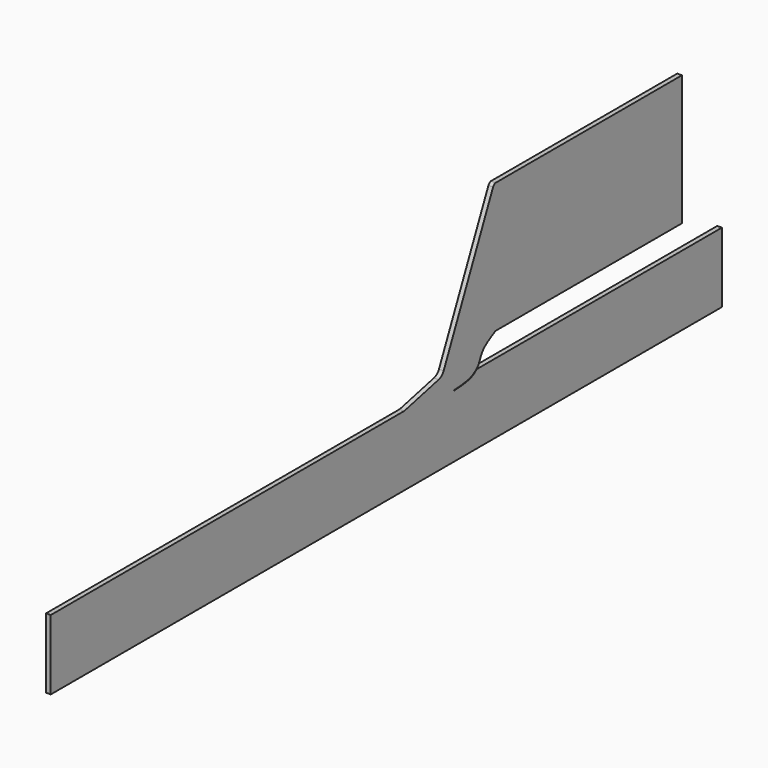
from build123d import *

# Parameters (mm, degrees)
F0_W      = 1000
F0_H      = 150
F1_DEPTH  = 1800
F5_DEPTH  = 250
F7_DEPTH  = 250
F8_W      = 1814.4553899765
F8_H      = 676.3893961906
F9_DEPTH  = 500
F10_DEPTH = 500
F11_W     = 1876.0774359107
F11_H     = 584.96324718
F12_DEPTH = 490


# Not quite as in the source:
# - the dataset's text gives a spline's control points without its knots; the knots are read off the source's solid


with BuildPart() as f1:
    # F0 (on Front) → F1 (new body)
    with BuildSketch(Plane.XZ):
        with Locations((427.8578534722, -75)):
            Rectangle(F0_W, F0_H)
    extrude(amount=F1_DEPTH)

    # F4 (on plane+point) → F5 (join, symmetric)
    with BuildSketch(Plane.YZ.offset(427.8578534722)):
        with BuildLine():
            add(Edge.make_bspline(
                [(-658.5119275224, 0), (-663.1096709351, -3.3994040102), (-674.8923410513, -12.2269214906), (-701.8084297627, -13.9660228128), (-718.060195446, -15.0110442191)],
                knots=[0, 0, 0, 0, 0.3960668718, 1, 1, 1, 1], degree=3))
            add(Edge.make_bspline(
                [(-658.5119275224, 0), (-650.3595915647, 6.0275402647), (-648.0235359943, 31.4958112046), (-617.163744576, 46.1983191108), (-607.3494242193, 51.7760817812)],
                knots=[0, 0, 0, 0, 0.4646733695, 1, 1, 1, 1], degree=3))
            Line((-607.3494242193, 51.7760817812), (-607.3494242193, 331.3955929823))
            ThreePointArc((-607.3494242193, 331.3955929823), (-611.1459562468, 329.3507401392), (-613.7284624486, 325.8973736217))
            Line((-613.7284624486, 325.8973736217), (-746.2776173449, 32.8608466306))
            ThreePointArc((-746.2776173449, 32.8608466306), (-751.7911260188, 25.6605897485), (-759.9176837495, 21.6354765186))
            Line((-759.9176837495, 21.6354765186), (-851.8334031105, 0))
            Line((-851.8334031105, 0), (-724.4437932968, 0))
            Line((-724.4437932968, 0), (-718.060195446, -15.0110442191))
        make_face()
    extrude(amount=F5_DEPTH, both=True)

    # F6 (on plane+point) → F7 (cut, symmetric)
    with BuildSketch(Plane.YZ.offset(427.8578534722)):
        with BuildLine():
            add(Edge.make_bspline(
                [(-657.9174152342, -0.8040865247), (-659.3673865445, -1.8761424975), (-662.3030933204, -4.0564869069), (-666.4204873665, -6.6707717939), (-670.1931092733, -8.5651184529), (-673.3105086069, -9.8565410415), (-676.7740170416, -10.9816784698), (-681.8145421149, -12.2587633506), (-688.8193216778, -13.5004768766), (-698.0763714753, -14.5692911085), (-707.8993120937, -15.3593398489), (-714.632248917, -15.792685566), (-717.9960259489, -16.0089832331)],
                knots=[0, 0, 0, 0, 0.125, 0.25, 0.3125, 0.375, 0.4375, 0.5, 0.625, 0.75, 0.875, 1, 1, 1, 1], degree=3))
            Line((-657.9174152342, -0.8040865247), (-656.8298765035, 0))
            Line((-656.8298765035, 0), (-658.5119275224, 0))
            add(Edge.make_bspline(
                [(-658.5119275224, 0), (-663.1096709351, -3.3994040102), (-674.8923410513, -12.2269214906), (-701.8084297627, -13.9660228128), (-718.060195446, -15.0110442191)],
                knots=[0, 0, 0, 0, 0.3960668718, 1, 1, 1, 1], degree=3))
            Line((-718.060195446, -15.0110442191), (-717.9960259489, -16.0089832331))
        make_face()
    extrude(amount=F7_DEPTH, both=True, mode=Mode.SUBTRACT)

    # F8 (on plane+point) → F9 (cut, through all)
    with BuildSketch(Plane.YZ.offset(427.8578534722)):
        with Locations((-907.2276949883, 182.6078593731)):
            Rectangle(F8_W, F8_H)
    extrude(amount=F9_DEPTH, mode=Mode.SUBTRACT)

    # F10 (add): a face of the model
    f10_faces = [f1.faces().sort_by_distance(p)[0] for p in [
        (302.8578534722, -607.3494242193, 191.5858373818),
    ]]
    extrude(f10_faces, amount=F10_DEPTH)

    # F11 (on face) → F12 (cut)
    with BuildSketch(Plane(origin=(-72.1421465278, 0, 0), x_dir=(0, -1, 0), z_dir=(-1, 0, 0))):
        with Locations((910.4874022305, 71.823425591)):
            Rectangle(F11_W, F11_H)
    extrude(amount=-F12_DEPTH, mode=Mode.SUBTRACT)


solid = f1.part
